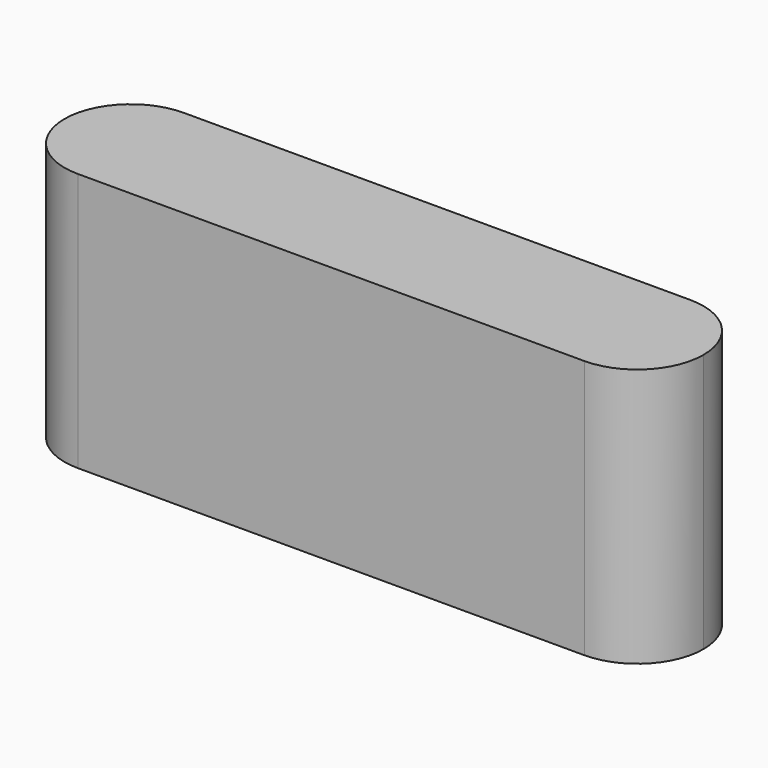
from build123d import *

# Parameters (mm, degrees)
F0_W     = 111
F0_H     = 45
F1_DEPTH = 11.5
F2_R     = 11.49999


# Not quite as in the source:
# - a fillet or chamfer is up to 0.001 mm smaller than in the source, because OpenCascade refuses the exact size


with BuildPart() as f1:
    # F0 (on Front) → F1 (new body, symmetric)
    with BuildSketch(Plane.XZ):
        Rectangle(F0_W, F0_H)
    extrude(amount=F1_DEPTH, both=True)

    # F2 (radius 11.5 in the source; OpenCascade refuses exactly that, so slightly less here)
    f2_edges = [f1.edges().sort_by_distance(p)[0] for p in [
        (-55.5, -11.5, 0),
        (-55.5, 11.5, 0),
        (55.5, 11.5, 0),
        (55.5, -11.5, 0),
    ]]
    fillet(f2_edges, radius=F2_R)


solid = f1.part
